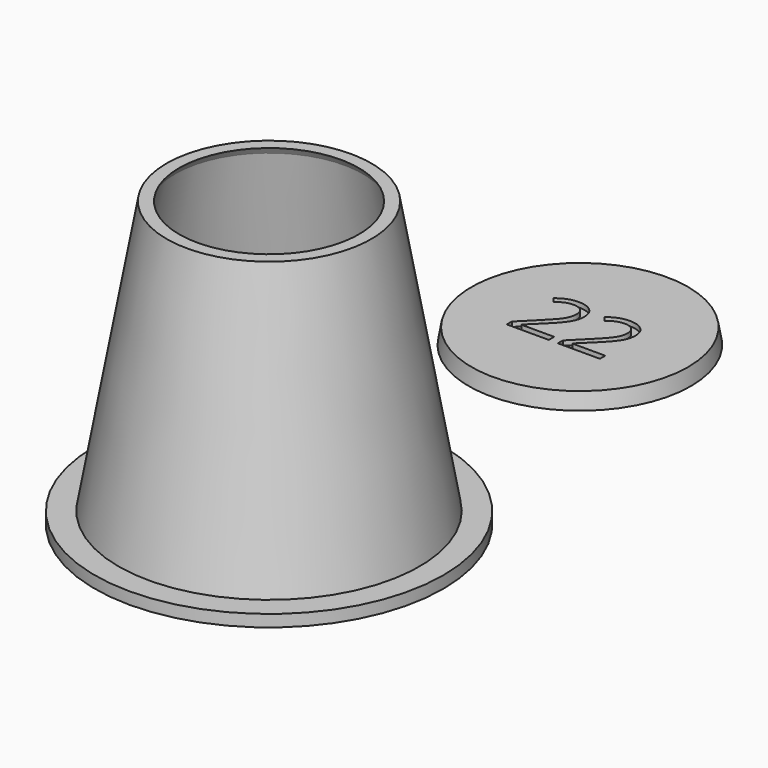
from build123d import *

# Parameters (mm, degrees)
F2_R         = 14
F3_DEPTH     = 2
F3_TAPER     = 10
F2_R_2       = 12
F4_TEXT_SIZE = 11.2402053499
F5_TEXT_SIZE = 11.2584573748
F6_DEPTH     = 0.6


# Not quite as in the source:
# - Text() gives the source's letters only with a copy of the font that has no kerning and outlines rounded to 1/6400 em; it was checked with that copy


with BuildPart() as f1:
    # F0 (on Front) → F1 (revolve)
    with BuildSketch(Plane.XZ):
        Polygon((-18, 0), (-11.8285556752, 35), (-11.3151815206, 35.8395585988), (-12.8990307766, 35.8395585988), (-18.9540214632, 1.5), (-21.9540214632, 1.5), (-21.9540214632, 0), align=None)
    revolve(axis=Axis((0, 0, 17.5), (0, 0, 1)))


with BuildPart() as f3:
    # F2 (on Top) → F3 (new body)
    with BuildSketch(Plane.XY):
        with Locations((0, 48.9216328317)):
            Circle(F2_R)
    extrude(amount=F3_DEPTH, taper=F3_TAPER)


with BuildPart() as f3b:
    # F2 (on Top) → F3, piece 2 (new body)
    with BuildSketch(Plane.XY):
        with Locations((-38.3968576789, 48.9216328317)):
            Circle(F2_R_2)
    extrude(amount=F3_DEPTH, taper=F3_TAPER)


with BuildPart() as f6_tool:
    # F4 (on face) + F5 (on face) → F6 (new body)
    with BuildSketch(Plane.XY.offset(2)):
        with Locations((-44.8968576789, 44.8751589057)):
            Text('28', F4_TEXT_SIZE, font='Open Sans', text_align=(TextAlign.LEFT, TextAlign.BOTTOM))
    with BuildSketch(Plane.XY.offset(2)):
        with Locations((-6.5, 44.8685881768)):
            Text('22', F5_TEXT_SIZE, font='Open Sans', text_align=(TextAlign.LEFT, TextAlign.BOTTOM))
    extrude(amount=-F6_DEPTH)


with BuildPart() as f3_1:
    add(f3.part)

    # F6: cut by f6_tool
    add(f6_tool.part, mode=Mode.SUBTRACT)


with BuildPart() as f3b_1:
    add(f3b.part)

    # F6: cut by f6_tool
    add(f6_tool.part, mode=Mode.SUBTRACT)


solid = Compound([f1.part, f3_1.part, f3b_1.part])
